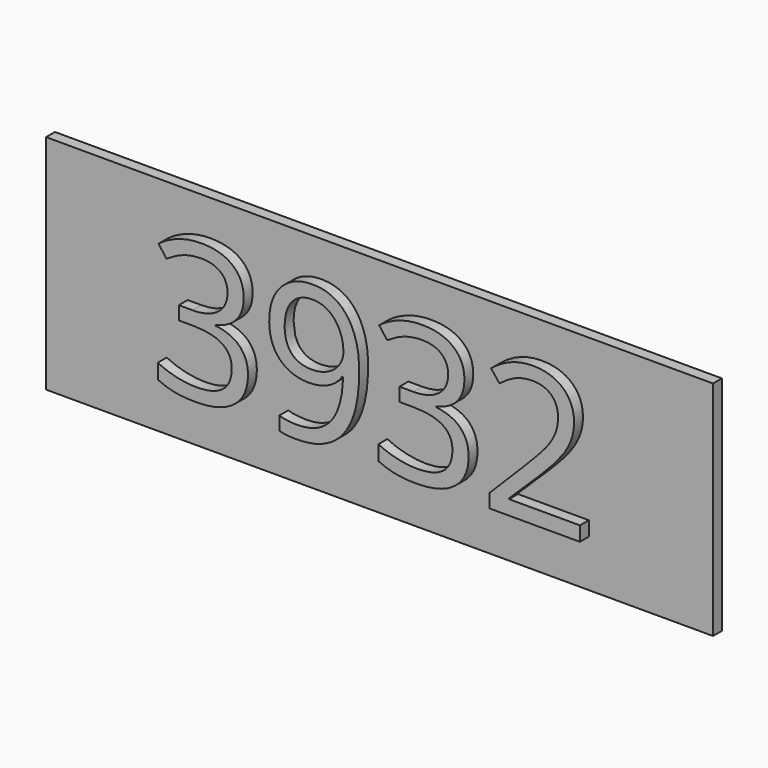
from build123d import *

# Parameters (mm, degrees)
F0_TEXT_SIZE = 88.1944444444
F1_DEPTH     = 10.16
F0_W         = 304.8
F0_H         = 101.6
F2_DEPTH     = 5.08


# Not quite as in the source:
# - Text() gives the source's letters only with a copy of the font that has no kerning and outlines rounded to 1/6400 em; it was checked with that copy


with BuildPart() as f1:
    # F0 (on Front) → F1 (new body)
    with BuildSketch(Plane.XZ):
        with Locations((-101.3409288194, -29.3009031207)):
            Text('3932', F0_TEXT_SIZE, font='Open Sans', text_align=(TextAlign.LEFT, TextAlign.BOTTOM))
    extrude(amount=F1_DEPTH)


with BuildPart() as f2:
    # F0 (on Front) → F2 (new body)
    with BuildSketch(Plane.XZ):
        Rectangle(F0_W, F0_H)
        with BuildLine():
            add(Edge.make_bspline(
                [(-63.1003689236, 30.3612605077), (-58.0154079861, 26.1651342056), (-58.0154079861, 18.8477513931)],
                knots=[0, 0, 0, 1, 1, 1], degree=2))
            add(Edge.make_bspline(
                [(-58.0154079861, 18.8477513931), (-58.0154079861, 12.8119441015), (-61.3984917535, 8.9809979209)],
                knots=[0, 0, 0, 1, 1, 1], degree=2))
            add(Edge.make_bspline(
                [(-61.3984917535, 8.9809979209), (-64.7815755208, 5.1500517404), (-70.9827473958, 3.8546958376)],
                knots=[0, 0, 0, 1, 1, 1], degree=2))
            Line((-70.9827473958, 3.8546958376), (-70.9827473958, 3.510186289))
            add(Edge.make_bspline(
                [(-70.9827473958, 3.510186289), (-63.4035373264, 2.5731203168), (-59.7448459201, -1.3060572006)],
                knots=[0, 0, 0, 1, 1, 1], degree=2))
            add(Edge.make_bspline(
                [(-59.7448459201, -1.3060572006), (-56.0861545139, -5.185234718), (-56.0861545139, -11.4690888846)],
                knots=[0, 0, 0, 1, 1, 1], degree=2))
            add(Edge.make_bspline(
                [(-56.0861545139, -11.4690888846), (-56.0861545139, -20.4676782944), (-62.3286675347, -25.3183727388)],
                knots=[0, 0, 0, 1, 1, 1], degree=2))
            add(Edge.make_bspline(
                [(-62.3286675347, -25.3183727388), (-68.5711805556, -30.1690671832), (-80.0640190972, -30.1690671832)],
                knots=[0, 0, 0, 1, 1, 1], degree=2))
            add(Edge.make_bspline(
                [(-80.0640190972, -30.1690671832), (-85.0662977431, -30.1690671832), (-89.2210828993, -29.4111461763)],
                knots=[0, 0, 0, 1, 1, 1], degree=2))
            add(Edge.make_bspline(
                [(-89.2210828993, -29.4111461763), (-93.3758680556, -28.6532251694), (-97.2894965278, -26.765312843)],
                knots=[0, 0, 0, 1, 1, 1], degree=2))
            Line((-97.2894965278, -26.765312843), (-97.2894965278, -19.9578041624))
            add(Edge.make_bspline(
                [(-97.2894965278, -19.9578041624), (-93.1967230903, -21.9835203082), (-88.5665147569, -23.037719527)],
                knots=[0, 0, 0, 1, 1, 1], degree=2))
            add(Edge.make_bspline(
                [(-88.5665147569, -23.037719527), (-83.9363064236, -24.0919187457), (-79.8021918403, -24.0919187457)],
                knots=[0, 0, 0, 1, 1, 1], degree=2))
            add(Edge.make_bspline(
                [(-79.8021918403, -24.0919187457), (-63.4862196181, -24.0919187457), (-63.4862196181, -11.3037243013)],
                knots=[0, 0, 0, 1, 1, 1], degree=2))
            add(Edge.make_bspline(
                [(-63.4862196181, -11.3037243013), (-63.4862196181, 0.1615534765), (-81.4833984375, 0.1615534765)],
                knots=[0, 0, 0, 1, 1, 1], degree=2))
            Line((-81.4833984375, 0.1615534765), (-87.6845703125, 0.1615534765))
            Line((-87.6845703125, 0.1615534765), (-87.6845703125, 6.3076038237))
            Line((-87.6845703125, 6.3076038237), (-81.4007161458, 6.3076038237))
            add(Edge.make_bspline(
                [(-81.4007161458, 6.3076038237), (-74.0419921875, 6.3076038237), (-69.7356228299, 9.5597739626)],
                knots=[0, 0, 0, 1, 1, 1], degree=2))
            add(Edge.make_bspline(
                [(-69.7356228299, 9.5597739626), (-65.4292534722, 12.8119441015), (-65.4292534722, 18.5859241362)],
                knots=[0, 0, 0, 1, 1, 1], degree=2))
            add(Edge.make_bspline(
                [(-65.4292534722, 18.5859241362), (-65.4292534722, 23.1885717056), (-68.5918511285, 25.820624657)],
                knots=[0, 0, 0, 1, 1, 1], degree=2))
            add(Edge.make_bspline(
                [(-68.5918511285, 25.820624657), (-71.7544487847, 28.4526776084), (-77.1839192708, 28.4526776084)],
                knots=[0, 0, 0, 1, 1, 1], degree=2))
            add(Edge.make_bspline(
                [(-77.1839192708, 28.4526776084), (-81.3180338542, 28.4526776084), (-84.9767252604, 27.3295764799)],
                knots=[0, 0, 0, 1, 1, 1], degree=2))
            add(Edge.make_bspline(
                [(-84.9767252604, 27.3295764799), (-88.6354166667, 26.2064753515), (-93.3345269097, 23.1885717056)],
                knots=[0, 0, 0, 1, 1, 1], degree=2))
            Line((-93.3345269097, 23.1885717056), (-96.9449869792, 28.0117053862))
            add(Edge.make_bspline(
                [(-96.9449869792, 28.0117053862), (-93.0726996528, 31.0709501779), (-88.0152994792, 32.8141684938)],
                knots=[0, 0, 0, 1, 1, 1], degree=2))
            add(Edge.make_bspline(
                [(-88.0152994792, 32.8141684938), (-82.9578993056, 34.5573868098), (-77.3492838542, 34.5573868098)],
                knots=[0, 0, 0, 1, 1, 1], degree=2))
            add(Edge.make_bspline(
                [(-77.3492838542, 34.5573868098), (-68.1853298611, 34.5573868098), (-63.1003689236, 30.3612605077)],
                knots=[0, 0, 0, 1, 1, 1], degree=2))
        make_face(mode=Mode.SUBTRACT)
        with BuildLine():
            add(Edge.make_bspline(
                [(-7.8065863715, 21.6658395008), (-5.2227647569, 15.3613147612), (-5.2227647569, 6.7899171918)],
                knots=[0, 0, 0, 1, 1, 1], degree=2))
            add(Edge.make_bspline(
                [(-5.2227647569, 6.7899171918), (-5.2227647569, -30.1690671832), (-33.8170572917, -30.1690671832)],
                knots=[0, 0, 0, 1, 1, 1], degree=2))
            add(Edge.make_bspline(
                [(-33.8170572917, -30.1690671832), (-38.8193359375, -30.1690671832), (-41.7407769097, -29.3009031207)],
                knots=[0, 0, 0, 1, 1, 1], degree=2))
            Line((-41.7407769097, -29.3009031207), (-41.7407769097, -23.1410723916))
            add(Edge.make_bspline(
                [(-41.7407769097, -23.1410723916), (-38.2956814236, -24.2572833291), (-33.9135199653, -24.2572833291)],
                knots=[0, 0, 0, 1, 1, 1], degree=2))
            add(Edge.make_bspline(
                [(-33.9135199653, -24.2572833291), (-23.5782335069, -24.2572833291), (-18.3003472222, -17.8631861069)],
                knots=[0, 0, 0, 1, 1, 1], degree=2))
            add(Edge.make_bspline(
                [(-18.3003472222, -17.8631861069), (-13.0224609375, -11.4690888846), (-12.5539279514, 1.7462974001)],
                knots=[0, 0, 0, 1, 1, 1], degree=2))
            Line((-12.5539279514, 1.7462974001), (-13.0638020833, 1.7462974001))
            add(Edge.make_bspline(
                [(-13.0638020833, 1.7462974001), (-15.4340277778, -1.8228215235), (-19.354546441, -3.696953468)],
                knots=[0, 0, 0, 1, 1, 1], degree=2))
            add(Edge.make_bspline(
                [(-19.354546441, -3.696953468), (-23.2750651042, -5.5710854124), (-28.1808810764, -5.5710854124)],
                knots=[0, 0, 0, 1, 1, 1], degree=2))
            add(Edge.make_bspline(
                [(-28.1808810764, -5.5710854124), (-36.5317925347, -5.5710854124), (-41.4444986979, -0.5756969576)],
                knots=[0, 0, 0, 1, 1, 1], degree=2))
            add(Edge.make_bspline(
                [(-41.4444986979, -0.5756969576), (-46.3572048611, 4.4196914973), (-46.3572048611, 13.3769397612)],
                knots=[0, 0, 0, 1, 1, 1], degree=2))
            add(Edge.make_bspline(
                [(-46.3572048611, 13.3769397612), (-46.3572048611, 23.1885717056), (-40.8657226563, 28.8729792577)],
                knots=[0, 0, 0, 1, 1, 1], degree=2))
            add(Edge.make_bspline(
                [(-40.8657226563, 28.8729792577), (-35.3742404514, 34.5573868098), (-26.4169921875, 34.5573868098)],
                knots=[0, 0, 0, 1, 1, 1], degree=2))
            add(Edge.make_bspline(
                [(-26.4169921875, 34.5573868098), (-19.9953342014, 34.5573868098), (-15.1928710938, 31.2638755251)],
                knots=[0, 0, 0, 1, 1, 1], degree=2))
            add(Edge.make_bspline(
                [(-15.1928710938, 31.2638755251), (-10.3904079861, 27.9703642404), (-7.8065863715, 21.6658395008)],
                knots=[0, 0, 0, 1, 1, 1], degree=2))
        make_face(mode=Mode.SUBTRACT)
        with BuildLine():
            add(Edge.make_bspline(
                [(37.7444661458, 30.3612605077), (42.8294270833, 26.1651342056), (42.8294270833, 18.8477513931)],
                knots=[0, 0, 0, 1, 1, 1], degree=2))
            add(Edge.make_bspline(
                [(42.8294270833, 18.8477513931), (42.8294270833, 12.8119441015), (39.446343316, 8.9809979209)],
                knots=[0, 0, 0, 1, 1, 1], degree=2))
            add(Edge.make_bspline(
                [(39.446343316, 8.9809979209), (36.0632595486, 5.1500517404), (29.8620876736, 3.8546958376)],
                knots=[0, 0, 0, 1, 1, 1], degree=2))
            Line((29.8620876736, 3.8546958376), (29.8620876736, 3.510186289))
            add(Edge.make_bspline(
                [(29.8620876736, 3.510186289), (37.4412977431, 2.5731203168), (41.0999891493, -1.3060572006)],
                knots=[0, 0, 0, 1, 1, 1], degree=2))
            add(Edge.make_bspline(
                [(41.0999891493, -1.3060572006), (44.7586805556, -5.185234718), (44.7586805556, -11.4690888846)],
                knots=[0, 0, 0, 1, 1, 1], degree=2))
            add(Edge.make_bspline(
                [(44.7586805556, -11.4690888846), (44.7586805556, -20.4676782944), (38.5161675347, -25.3183727388)],
                knots=[0, 0, 0, 1, 1, 1], degree=2))
            add(Edge.make_bspline(
                [(38.5161675347, -25.3183727388), (32.2736545139, -30.1690671832), (20.7808159722, -30.1690671832)],
                knots=[0, 0, 0, 1, 1, 1], degree=2))
            add(Edge.make_bspline(
                [(20.7808159722, -30.1690671832), (15.7785373264, -30.1690671832), (11.6237521701, -29.4111461763)],
                knots=[0, 0, 0, 1, 1, 1], degree=2))
            add(Edge.make_bspline(
                [(11.6237521701, -29.4111461763), (7.4689670139, -28.6532251694), (3.5553385417, -26.765312843)],
                knots=[0, 0, 0, 1, 1, 1], degree=2))
            Line((3.5553385417, -26.765312843), (3.5553385417, -19.9578041624))
            add(Edge.make_bspline(
                [(3.5553385417, -19.9578041624), (7.6481119792, -21.9835203082), (12.2783203125, -23.037719527)],
                knots=[0, 0, 0, 1, 1, 1], degree=2))
            add(Edge.make_bspline(
                [(12.2783203125, -23.037719527), (16.9085286458, -24.0919187457), (21.0426432292, -24.0919187457)],
                knots=[0, 0, 0, 1, 1, 1], degree=2))
            add(Edge.make_bspline(
                [(21.0426432292, -24.0919187457), (37.3586154514, -24.0919187457), (37.3586154514, -11.3037243013)],
                knots=[0, 0, 0, 1, 1, 1], degree=2))
            add(Edge.make_bspline(
                [(37.3586154514, -11.3037243013), (37.3586154514, 0.1615534765), (19.3614366319, 0.1615534765)],
                knots=[0, 0, 0, 1, 1, 1], degree=2))
            Line((19.3614366319, 0.1615534765), (13.1602647569, 0.1615534765))
            Line((13.1602647569, 0.1615534765), (13.1602647569, 6.3076038237))
            Line((13.1602647569, 6.3076038237), (19.4441189236, 6.3076038237))
            add(Edge.make_bspline(
                [(19.4441189236, 6.3076038237), (26.8028428819, 6.3076038237), (31.1092122396, 9.5597739626)],
                knots=[0, 0, 0, 1, 1, 1], degree=2))
            add(Edge.make_bspline(
                [(31.1092122396, 9.5597739626), (35.4155815972, 12.8119441015), (35.4155815972, 18.5859241362)],
                knots=[0, 0, 0, 1, 1, 1], degree=2))
            add(Edge.make_bspline(
                [(35.4155815972, 18.5859241362), (35.4155815972, 23.1885717056), (32.252983941, 25.820624657)],
                knots=[0, 0, 0, 1, 1, 1], degree=2))
            add(Edge.make_bspline(
                [(32.252983941, 25.820624657), (29.0903862847, 28.4526776084), (23.6609157986, 28.4526776084)],
                knots=[0, 0, 0, 1, 1, 1], degree=2))
            add(Edge.make_bspline(
                [(23.6609157986, 28.4526776084), (19.5268012153, 28.4526776084), (15.868109809, 27.3295764799)],
                knots=[0, 0, 0, 1, 1, 1], degree=2))
            add(Edge.make_bspline(
                [(15.868109809, 27.3295764799), (12.2094184028, 26.2064753515), (7.5103081597, 23.1885717056)],
                knots=[0, 0, 0, 1, 1, 1], degree=2))
            Line((7.5103081597, 23.1885717056), (3.8998480903, 28.0117053862))
            add(Edge.make_bspline(
                [(3.8998480903, 28.0117053862), (7.7721354167, 31.0709501779), (12.8295355903, 32.8141684938)],
                knots=[0, 0, 0, 1, 1, 1], degree=2))
            add(Edge.make_bspline(
                [(12.8295355903, 32.8141684938), (17.8869357639, 34.5573868098), (23.4955512153, 34.5573868098)],
                knots=[0, 0, 0, 1, 1, 1], degree=2))
            add(Edge.make_bspline(
                [(23.4955512153, 34.5573868098), (32.6595052083, 34.5573868098), (37.7444661458, 30.3612605077)],
                knots=[0, 0, 0, 1, 1, 1], degree=2))
        make_face(mode=Mode.SUBTRACT)
        with BuildLine():
            Line((95.6220703125, -22.6725394055), (95.6220703125, -29.3009031207))
            Line((95.6220703125, -29.3009031207), (54.2395833333, -29.3009031207))
            Line((54.2395833333, -29.3009031207), (54.2395833333, -23.1410723916))
            Line((54.2395833333, -23.1410723916), (70.8173828125, -6.4805906207))
            add(Edge.make_bspline(
                [(70.8173828125, -6.4805906207), (78.3965928819, 1.1950821223), (80.8081597222, 4.4679228341)],
                knots=[0, 0, 0, 1, 1, 1], degree=2))
            add(Edge.make_bspline(
                [(80.8081597222, 4.4679228341), (83.2197265625, 7.7407635459), (84.4255099826, 10.8413494834)],
                knots=[0, 0, 0, 1, 1, 1], degree=2))
            add(Edge.make_bspline(
                [(84.4255099826, 10.8413494834), (85.6312934028, 13.9419354209), (85.6312934028, 17.5110543445)],
                knots=[0, 0, 0, 1, 1, 1], degree=2))
            add(Edge.make_bspline(
                [(85.6312934028, 17.5110543445), (85.6312934028, 22.5546741362), (82.5720486111, 25.5036758723)],
                knots=[0, 0, 0, 1, 1, 1], degree=2))
            add(Edge.make_bspline(
                [(82.5720486111, 25.5036758723), (79.5128038194, 28.4526776084), (74.0833333333, 28.4526776084)],
                knots=[0, 0, 0, 1, 1, 1], degree=2))
            add(Edge.make_bspline(
                [(74.0833333333, 28.4526776084), (70.1697048611, 28.4526776084), (66.6557074653, 27.1573217056)],
                knots=[0, 0, 0, 1, 1, 1], degree=2))
            add(Edge.make_bspline(
                [(66.6557074653, 27.1573217056), (63.1417100694, 25.8619658029), (58.8422309028, 22.4582114626)],
                knots=[0, 0, 0, 1, 1, 1], degree=2))
            Line((58.8422309028, 22.4582114626), (55.0526258681, 27.322686289))
            add(Edge.make_bspline(
                [(55.0526258681, 27.322686289), (63.748046875, 34.5573868098), (74.0006510417, 34.5573868098)],
                knots=[0, 0, 0, 1, 1, 1], degree=2))
            add(Edge.make_bspline(
                [(74.0006510417, 34.5573868098), (82.8752170139, 34.5573868098), (87.9119466146, 30.0167509591)],
                knots=[0, 0, 0, 1, 1, 1], degree=2))
            add(Edge.make_bspline(
                [(87.9119466146, 30.0167509591), (92.9486762153, 25.4761151084), (92.9486762153, 17.8142227473)],
                knots=[0, 0, 0, 1, 1, 1], degree=2))
            add(Edge.make_bspline(
                [(92.9486762153, 17.8142227473), (92.9486762153, 11.8197566015), (89.5862630208, 5.9630942751)],
                knots=[0, 0, 0, 1, 1, 1], degree=2))
            add(Edge.make_bspline(
                [(89.5862630208, 5.9630942751), (86.2238498264, 0.1064319487), (77.0185546875, -8.8508163152)],
                knots=[0, 0, 0, 1, 1, 1], degree=2))
            Line((77.0185546875, -8.8508163152), (63.2381727431, -22.3280298569))
            Line((63.2381727431, -22.3280298569), (63.2381727431, -22.6725394055))
            Line((63.2381727431, -22.6725394055), (95.6220703125, -22.6725394055))
        make_face(mode=Mode.SUBTRACT)
    extrude(amount=F2_DEPTH)


with BuildPart() as f2b:
    # F0 (on Front) → F2, piece 2 (new body)
    with BuildSketch(Plane.XZ):
        with BuildLine():
            add(Edge.make_bspline(
                [(-19.1616210938, 26.2547066883), (-22.32421875, 28.4526776084), (-26.4169921875, 28.4526776084)],
                knots=[0, 0, 0, 1, 1, 1], degree=2))
            add(Edge.make_bspline(
                [(-26.4169921875, 28.4526776084), (-32.5768229167, 28.4526776084), (-35.9323459201, 24.4908177994)],
                knots=[0, 0, 0, 1, 1, 1], degree=2))
            add(Edge.make_bspline(
                [(-35.9323459201, 24.4908177994), (-39.2878689236, 20.5289579904), (-39.2878689236, 13.4596220529)],
                knots=[0, 0, 0, 1, 1, 1], degree=2))
            add(Edge.make_bspline(
                [(-39.2878689236, 13.4596220529), (-39.2878689236, 7.2584501779), (-36.1872829861, 3.7100018272)],
                knots=[0, 0, 0, 1, 1, 1], degree=2))
            add(Edge.make_bspline(
                [(-36.1872829861, 3.7100018272), (-33.0866970486, 0.1615534765), (-26.7615017361, 0.1615534765)],
                knots=[0, 0, 0, 1, 1, 1], degree=2))
            add(Edge.make_bspline(
                [(-26.7615017361, 0.1615534765), (-22.8340928819, 0.1615534765), (-19.5405815972, 1.7531875911)],
                knots=[0, 0, 0, 1, 1, 1], degree=2))
            add(Edge.make_bspline(
                [(-19.5405815972, 1.7531875911), (-16.2470703125, 3.3448217056), (-14.3522677951, 6.1008980945)],
                knots=[0, 0, 0, 1, 1, 1], degree=2))
            add(Edge.make_bspline(
                [(-14.3522677951, 6.1008980945), (-12.4574652778, 8.8569744834), (-12.4574652778, 11.8748781293)],
                knots=[0, 0, 0, 1, 1, 1], degree=2))
            add(Edge.make_bspline(
                [(-12.4574652778, 11.8748781293), (-12.4574652778, 16.394843407), (-14.2282443576, 20.2257895876)],
                knots=[0, 0, 0, 1, 1, 1], degree=2))
            add(Edge.make_bspline(
                [(-14.2282443576, 20.2257895876), (-15.9990234375, 24.0567357681), (-19.1616210938, 26.2547066883)],
                knots=[0, 0, 0, 1, 1, 1], degree=2))
        make_face()
    extrude(amount=F2_DEPTH)


solid = Compound([f1.part, f2.part, f2b.part])
